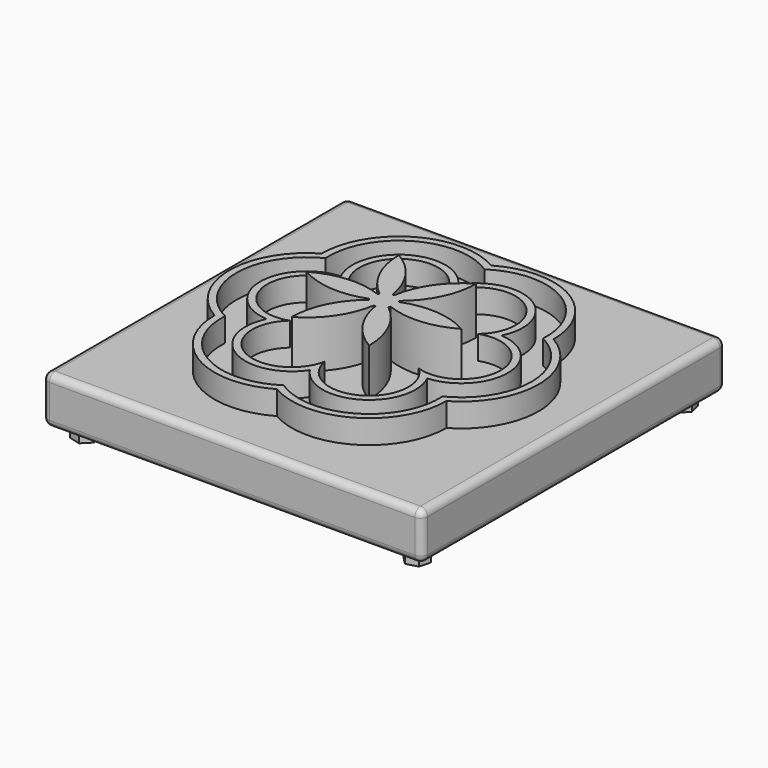
from build123d import *

# Parameters (mm, degrees)
F0_W     = 203.2
F0_H     = 203.2
F1_DEPTH = 25.4
F3_DEPTH = 6.35
F2_W     = 152.4
F2_H     = 152.4
F4_DEPTH = 6.35
F6_DEPTH = 12.7
F7_DEPTH = 12.7
F8_DEPTH = 12.7
F9_DEPTH = 12.7
F10_R    = 3.81


# Not quite as in the source:
# - a feature names something its author has since deleted; it is built from what else it names


with BuildPart() as f1:
    # F0 (on Top) → F1 (new body)
    with BuildSketch(Plane.XY):
        Rectangle(F0_W, F0_H)
    extrude(amount=F1_DEPTH)

    # F2 (on face) → F3 (join)
    with BuildSketch(Plane(origin=(0, 0, 0), x_dir=(1, 0, 0), z_dir=(0, 0, -1))):
        Polygon((-84.4098719395, -84.4098719395), (-90.5435009364, -82.7663710031), (-95.0336289969, -87.2564990636), (-93.3901280605, -93.3901280605), (-87.2564990636, -95.0336289969), (-82.7663710031, -90.5435009364), align=None)
        Polygon((90.5435009364, -82.7663710031), (84.4098719395, -84.4098719395), (82.7663710031, -90.5435009364), (87.2564990636, -95.0336289969), (93.3901280605, -93.3901280605), (95.0336289969, -87.2564990636), align=None)
        Polygon((93.3901280605, 93.3901280605), (87.2564990636, 95.0336289969), (82.7663710031, 90.5435009364), (84.4098719395, 84.4098719395), (90.5435009364, 82.7663710031), (95.0336289969, 87.2564990636), align=None)
        Polygon((-95.0336289969, 87.2564990636), (-90.5435009364, 82.7663710031), (-84.4098719395, 84.4098719395), (-82.7663710031, 90.5435009364), (-87.2564990636, 95.0336289969), (-93.3901280605, 93.3901280605), align=None)
    extrude(amount=F3_DEPTH)

    # F2 (on face) → F4 (join)
    with BuildSketch(Plane(origin=(0, 0, 0), x_dir=(1, 0, 0), z_dir=(0, 0, -1))):
        Rectangle(F2_W, F2_H)
    extrude(amount=F4_DEPTH)

    # F5 (on face) → F6 (join)
    with BuildSketch(Plane.XY.offset(25.4)):
        with BuildLine():
            ThreePointArc((0, -71.685720599), (41.3877700849, -71.685720599), (62.0816551274, -35.8428602995))
            ThreePointArc((62.0816551274, -35.8428602995), (82.7755401698, 0), (62.0816551274, 35.8428602995))
            ThreePointArc((62.0816551274, 35.8428602995), (41.3877700849, 71.685720599), (0, 71.685720599))
            ThreePointArc((0, 71.685720599), (-41.3877700849, 71.685720599), (-62.0816551274, 35.8428602995))
            ThreePointArc((-62.0816551274, 35.8428602995), (-82.7755401698, 0), (-62.0816551274, -35.8428602995))
            ThreePointArc((-62.0816551274, -35.8428602995), (-41.3877700849, -71.685720599), (0, -71.685720599))
        make_face()
        with BuildLine():
            ThreePointArc((0, 67.2092742865), (39.4827700849, 68.3861638106), (58.204938902, 33.6046371433))
            ThreePointArc((58.204938902, 33.6046371433), (78.9655401698, 0), (58.204938902, -33.6046371433))
            ThreePointArc((58.204938902, -33.6046371433), (39.4827700849, -68.3861638106), (0, -67.2092742865))
            ThreePointArc((0, -67.2092742865), (-39.4827700849, -68.3861638106), (-58.204938902, -33.6046371433))
            ThreePointArc((-58.204938902, -33.6046371433), (-78.9655401698, 0), (-58.204938902, 33.6046371433))
            ThreePointArc((-58.204938902, 33.6046371433), (-39.4827700849, 68.3861638106), (0, 67.2092742865))
        make_face(mode=Mode.SUBTRACT)
    extrude(amount=F6_DEPTH)

    # F5 (on face) → F7 (join)
    with BuildSketch(Plane.XY.offset(25.4)):
        with BuildLine():
            ThreePointArc((42.9990851577, -24.8255333907), (66.2655401698, 0), (42.9990851577, 24.8255333907))
            ThreePointArc((42.9990851577, 24.8255333907), (33.1327700849, 57.3876411826), (0, 49.6510667814))
            ThreePointArc((0, 49.6510667814), (-33.1327700849, 57.3876411826), (-42.9990851577, 24.8255333907))
            ThreePointArc((-42.9990851577, 24.8255333907), (-66.2655401698, 0), (-42.9990851577, -24.8255333907))
            ThreePointArc((-42.9990851577, -24.8255333907), (-33.1327700849, -57.3876411826), (0, -49.6510667814))
            ThreePointArc((0, -49.6510667814), (33.1327700849, -57.3876411826), (42.9990851577, -24.8255333907))
        make_face()
        with BuildLine():
            ThreePointArc((-34.4628947241, 19.897161546), (-31.2277700849, 54.0880843941), (0, 39.794323092))
            ThreePointArc((0, 39.794323092), (31.2277700849, 54.0880843941), (34.4628947241, 19.897161546))
            ThreePointArc((34.4628947241, 19.897161546), (62.4555401698, 0), (34.4628947241, -19.897161546))
            ThreePointArc((34.4628947241, -19.897161546), (31.2277700849, -54.0880843941), (0, -39.794323092))
            ThreePointArc((0, -39.794323092), (-31.2277700849, -54.0880843941), (-34.4628947241, -19.897161546))
            ThreePointArc((-34.4628947241, -19.897161546), (-62.4555401698, 0), (-34.4628947241, 19.897161546))
        make_face(mode=Mode.SUBTRACT)
    extrude(amount=F7_DEPTH)

    # F5 (on face) → F8 (join)
    with BuildSketch(Plane.XY.offset(25.4)):
        with BuildLine():
            ThreePointArc((-5.2394906659, -3.5875113327), (-16.6308527593, -17.9595870916), (-20.6938850425, -35.8428602995))
            ThreePointArc((-20.6938850425, -35.8428602995), (-7.2380322831, -23.382534522), (-0.4871306175, -6.3312876859))
            ThreePointArc((-0.4871306175, -6.3312876859), (0, -6.35), (0.4871306175, -6.3312876859))
            ThreePointArc((0.4871306175, -6.3312876859), (7.2380322831, -23.382534522), (20.6938850425, -35.8428602995))
            ThreePointArc((20.6938850425, -35.8428602995), (16.6308527593, -17.9595870916), (5.2394906659, -3.5875113327))
            ThreePointArc((5.2394906659, -3.5875113327), (5.499261314, -3.175), (5.7266212834, -2.7437763532))
            ThreePointArc((5.7266212834, -2.7437763532), (23.8688850425, -5.4229474304), (41.3877700849, 0))
            ThreePointArc((41.3877700849, 0), (23.8688850425, 5.4229474304), (5.7266212834, 2.7437763532))
            ThreePointArc((5.7266212834, 2.7437763532), (5.499261314, 3.175), (5.2394906659, 3.5875113327))
            ThreePointArc((5.2394906659, 3.5875113327), (16.6308527593, 17.9595870916), (20.6938850425, 35.8428602995))
            ThreePointArc((20.6938850425, 35.8428602995), (7.2380322831, 23.382534522), (0.4871306175, 6.3312876859))
            ThreePointArc((0.4871306175, 6.3312876859), (0, 6.35), (-0.4871306175, 6.3312876859))
            ThreePointArc((-0.4871306175, 6.3312876859), (-7.2380322831, 23.382534522), (-20.6938850425, 35.8428602995))
            ThreePointArc((-20.6938850425, 35.8428602995), (-16.6308527593, 17.9595870916), (-5.2394906659, 3.5875113327))
            ThreePointArc((-5.2394906659, 3.5875113327), (-5.499261314, 3.175), (-5.7266212834, 2.7437763532))
            ThreePointArc((-5.7266212834, 2.7437763532), (-23.8688850425, 5.4229474304), (-41.3877700849, 0))
            ThreePointArc((-41.3877700849, 0), (-23.8688850425, -5.4229474304), (-5.7266212834, -2.7437763532))
            ThreePointArc((-5.7266212834, -2.7437763532), (-5.499261314, -3.175), (-5.2394906659, -3.5875113327))
        make_face()
    extrude(amount=F8_DEPTH)

    # F5 (on face) + F8_face (on face) → F9 (join)
    with BuildSketch(Plane.XY.offset(25.4)):
        with BuildLine():
            ThreePointArc((-5.2394906659, -3.5875113327), (-16.6308527593, -17.9595870916), (-20.6938850425, -35.8428602995))
            ThreePointArc((-20.6938850425, -35.8428602995), (-7.2380322831, -23.382534522), (-0.4871306175, -6.3312876859))
            ThreePointArc((-0.4871306175, -6.3312876859), (0, -6.35), (0.4871306175, -6.3312876859))
            ThreePointArc((0.4871306175, -6.3312876859), (7.2380322831, -23.382534522), (20.6938850425, -35.8428602995))
            ThreePointArc((20.6938850425, -35.8428602995), (16.6308527593, -17.9595870916), (5.2394906659, -3.5875113327))
            ThreePointArc((5.2394906659, -3.5875113327), (5.499261314, -3.175), (5.7266212834, -2.7437763532))
            ThreePointArc((5.7266212834, -2.7437763532), (23.8688850425, -5.4229474304), (41.3877700849, 0))
            ThreePointArc((41.3877700849, 0), (23.8688850425, 5.4229474304), (5.7266212834, 2.7437763532))
            ThreePointArc((5.7266212834, 2.7437763532), (5.499261314, 3.175), (5.2394906659, 3.5875113327))
            ThreePointArc((5.2394906659, 3.5875113327), (16.6308527593, 17.9595870916), (20.6938850425, 35.8428602995))
            ThreePointArc((20.6938850425, 35.8428602995), (7.2380322831, 23.382534522), (0.4871306175, 6.3312876859))
            ThreePointArc((0.4871306175, 6.3312876859), (0, 6.35), (-0.4871306175, 6.3312876859))
            ThreePointArc((-0.4871306175, 6.3312876859), (-7.2380322831, 23.382534522), (-20.6938850425, 35.8428602995))
            ThreePointArc((-20.6938850425, 35.8428602995), (-16.6308527593, 17.9595870916), (-5.2394906659, 3.5875113327))
            ThreePointArc((-5.2394906659, 3.5875113327), (-5.499261314, 3.175), (-5.7266212834, 2.7437763532))
            ThreePointArc((-5.7266212834, 2.7437763532), (-23.8688850425, 5.4229474304), (-41.3877700849, 0))
            ThreePointArc((-41.3877700849, 0), (-23.8688850425, -5.4229474304), (-5.7266212834, -2.7437763532))
            ThreePointArc((-5.7266212834, -2.7437763532), (-5.499261314, -3.175), (-5.2394906659, -3.5875113327))
        make_face()
    with BuildSketch(Plane.XY.offset(38.1)):
        with BuildLine():
            ThreePointArc((-5.7266212834, 2.7437763532), (-23.8688850425, 5.4229474304), (-41.3877700849, 0))
            ThreePointArc((-41.3877700849, 0), (-23.8688850425, -5.4229474304), (-5.7266212834, -2.7437763532))
            ThreePointArc((-5.7266212834, -2.7437763532), (-5.499261314, -3.175), (-5.2394906659, -3.5875113327))
            ThreePointArc((-5.2394906659, -3.5875113327), (-16.6308527593, -17.9595870916), (-20.6938850425, -35.8428602995))
            ThreePointArc((-20.6938850425, -35.8428602995), (-7.2380322831, -23.382534522), (-0.4871306175, -6.3312876859))
            ThreePointArc((-0.4871306175, -6.3312876859), (0, -6.35), (0.4871306175, -6.3312876859))
            ThreePointArc((0.4871306175, -6.3312876859), (7.2380322831, -23.382534522), (20.6938850425, -35.8428602995))
            ThreePointArc((20.6938850425, -35.8428602995), (16.6308527593, -17.9595870916), (5.2394906659, -3.5875113327))
            ThreePointArc((5.2394906659, -3.5875113327), (5.499261314, -3.175), (5.7266212834, -2.7437763532))
            ThreePointArc((5.7266212834, -2.7437763532), (23.8688850425, -5.4229474304), (41.3877700849, 0))
            ThreePointArc((41.3877700849, 0), (23.8688850425, 5.4229474304), (5.7266212834, 2.7437763532))
            ThreePointArc((5.7266212834, 2.7437763532), (5.499261314, 3.175), (5.2394906659, 3.5875113327))
            ThreePointArc((5.2394906659, 3.5875113327), (16.6308527593, 17.9595870916), (20.6938850425, 35.8428602995))
            ThreePointArc((20.6938850425, 35.8428602995), (7.2380322831, 23.382534522), (0.4871306175, 6.3312876859))
            ThreePointArc((0.4871306175, 6.3312876859), (0, 6.35), (-0.4871306175, 6.3312876859))
            ThreePointArc((-0.4871306175, 6.3312876859), (-7.2380322831, 23.382534522), (-20.6938850425, 35.8428602995))
            ThreePointArc((-20.6938850425, 35.8428602995), (-16.6308527593, 17.9595870916), (-5.2394906659, 3.5875113327))
            ThreePointArc((-5.2394906659, 3.5875113327), (-5.499261314, 3.175), (-5.7266212834, 2.7437763532))
        make_face()
    extrude(amount=F9_DEPTH)

    # F10
    f10_edges = [f1.edges().sort_by_distance(p)[0] for p in [
        (0, 101.6, 25.4),
        (-101.6, 0, 25.4),
        (101.6, 0, 25.4),
        (0, -101.6, 25.4),
        (101.6, 101.6, 12.7),
        (-101.6, 101.6, 12.7),
        (-101.6, -101.6, 12.7),
        (101.6, -101.6, 12.7),
        (101.6, 0, 0),
        (0, -101.6, 0),
        (-101.6, 0, 0),
        (0, 101.6, 0),
    ]]
    fillet(f10_edges, radius=F10_R)


solid = f1.part
